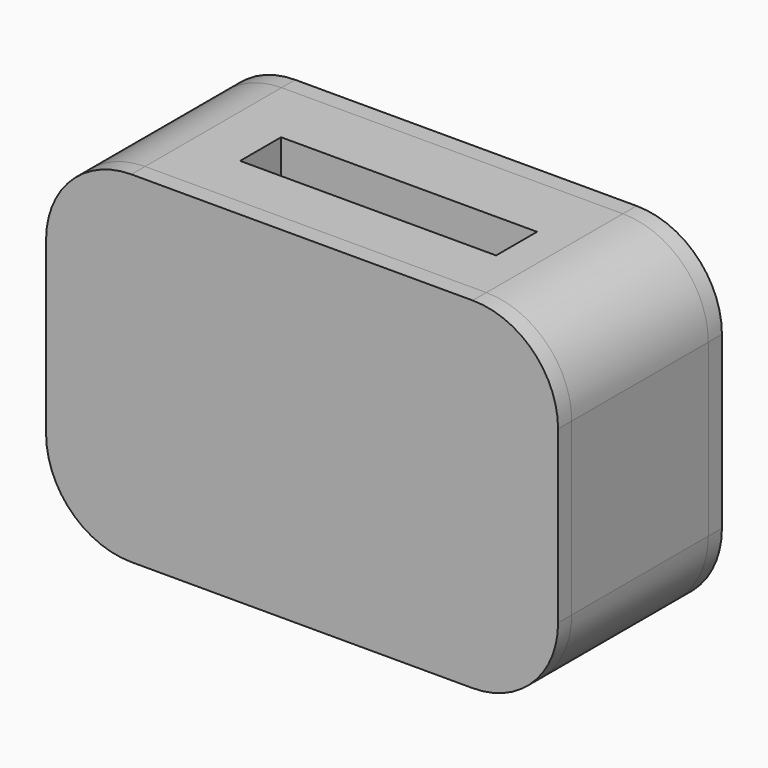
from build123d import *

# Parameters (mm, degrees)
F0_W      = 150
F0_H      = 100
F1_DEPTH  = 50
F2_DEPTH  = 5
F3_W      = 80
F3_H      = 40
F4_DEPTH  = 100
F5_W      = 150
F5_H      = 100
F6_DEPTH  = 5
F8_R      = 25
F9_R      = 25
F10_R     = 25
F11_R     = 25
F12_R     = 25
F13_R     = 25
F14_R     = 25
F15_R     = 25
F16_R     = 25
F17_R     = 25
F18_R     = 25
F19_R     = 25
F20_W     = 80
F20_H     = 40
F21_DEPTH = 100
F22_W     = 75
F22_H     = 15
F23_DEPTH = 80.9


with BuildPart() as f1:
    # F0 (on Front) → F1 (new body)
    with BuildSketch(Plane.XZ):
        Rectangle(F0_W, F0_H)
    extrude(amount=F1_DEPTH)


with BuildPart() as f2:
    # F2 (new): a face of the model
    f2_faces = [f1.part.faces().sort_by_distance(p)[0] for p in [
        (0, -50, 0),
    ]]
    extrude(f2_faces, amount=F2_DEPTH)

    # F12
    f12_edges = [f2.edges().sort_by_distance(p)[0] for p in [
        (-75, -52.5, 50),
    ]]
    fillet(f12_edges, radius=F12_R)

    # F13
    f13_edges = [f2.edges().sort_by_distance(p)[0] for p in [
        (75, -52.5, 50),
    ]]
    fillet(f13_edges, radius=F13_R)

    # F14
    f14_edges = [f2.edges().sort_by_distance(p)[0] for p in [
        (-75, -52.5, -50),
    ]]
    fillet(f14_edges, radius=F14_R)

    # F15
    f15_edges = [f2.edges().sort_by_distance(p)[0] for p in [
        (75, -52.5, -50),
    ]]
    fillet(f15_edges, radius=F15_R)


with BuildPart() as f1_1:
    add(f1.part)

    # F3 (on face) → F4 (cut)
    with BuildSketch(Plane(origin=(0, 0, 0), x_dir=(-1, 0, 0), z_dir=(0, 1, 0))):
        Rectangle(F3_W, F3_H)
    extrude(amount=-F4_DEPTH, mode=Mode.SUBTRACT)

    # F8
    f8_edges = [f1_1.edges().sort_by_distance(p)[0] for p in [
        (75, -25, 50),
    ]]
    fillet(f8_edges, radius=F8_R)

    # F9
    f9_edges = [f1_1.edges().sort_by_distance(p)[0] for p in [
        (-75, -25, 50),
    ]]
    fillet(f9_edges, radius=F9_R)

    # F10
    f10_edges = [f1_1.edges().sort_by_distance(p)[0] for p in [
        (-75, -25, -50),
    ]]
    fillet(f10_edges, radius=F10_R)

    # F11
    f11_edges = [f1_1.edges().sort_by_distance(p)[0] for p in [
        (75, -25, -50),
    ]]
    fillet(f11_edges, radius=F11_R)

    # F22 (on face) → F23 (cut)
    with BuildSketch(Plane.XY.offset(50)):
        with Locations((2.7394670993, -26.7461243272)):
            Rectangle(F22_W, F22_H)
    extrude(amount=-F23_DEPTH, mode=Mode.SUBTRACT)


with BuildPart() as f6:
    # F5 (on face) → F6 (new body)
    with BuildSketch(Plane(origin=(0, 0, 0), x_dir=(-1, 0, 0), z_dir=(0, 1, 0))):
        Rectangle(F5_W, F5_H)
    extrude(amount=F6_DEPTH)

    # F16
    f16_edges = [f6.edges().sort_by_distance(p)[0] for p in [
        (-75, 2.5, 50),
    ]]
    fillet(f16_edges, radius=F16_R)

    # F17
    f17_edges = [f6.edges().sort_by_distance(p)[0] for p in [
        (-75, 2.5, -50),
    ]]
    fillet(f17_edges, radius=F17_R)

    # F18
    f18_edges = [f6.edges().sort_by_distance(p)[0] for p in [
        (75, 2.5, 50),
    ]]
    fillet(f18_edges, radius=F18_R)

    # F19
    f19_edges = [f6.edges().sort_by_distance(p)[0] for p in [
        (75, 2.5, -50),
    ]]
    fillet(f19_edges, radius=F19_R)

    # F20 (on face) → F21 (cut)
    with BuildSketch(Plane(origin=(0, 5, 0), x_dir=(-1, 0, 0), z_dir=(0, 1, 0))):
        Rectangle(F20_W, F20_H)
    extrude(amount=-F21_DEPTH, mode=Mode.SUBTRACT)


solid = Compound([f2.part, f1_1.part, f6.part])
